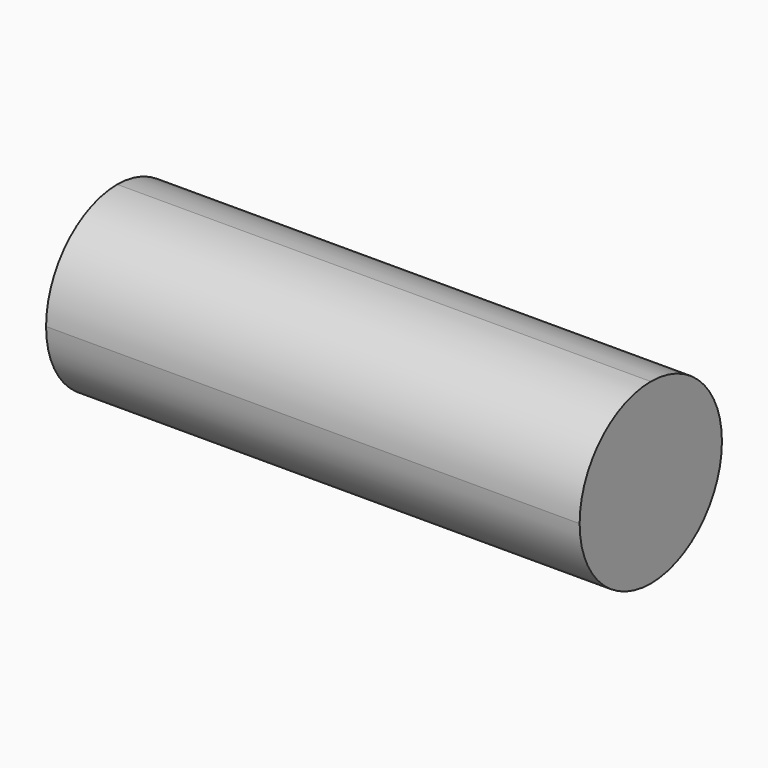
from build123d import *

# Parameters (mm, degrees)
F0_W     = 120
F0_H     = 40
F1_DEPTH = 40
F2_R     = 19.99999


# Not quite as in the source:
# - a fillet or chamfer is up to 0.001 mm smaller than in the source, because OpenCascade refuses the exact size


with BuildPart() as f1:
    # F0 (on Front) → F1 (new body)
    with BuildSketch(Plane.XZ):
        with Locations((-12.4206708372, 24.8193092685)):
            Rectangle(F0_W, F0_H)
    extrude(amount=F1_DEPTH)

    # F2 (radius 20 in the source; OpenCascade refuses exactly that, so slightly less here)
    f2_edges = [f1.edges().sort_by_distance(p)[0] for p in [
        (-12.420671, -40, 44.819309),
        (-12.420671, 0, 44.819309),
        (-12.420671, -40, 4.819309),
        (-12.420671, 0, 4.819309),
    ]]
    fillet(f2_edges, radius=F2_R)


solid = f1.part
